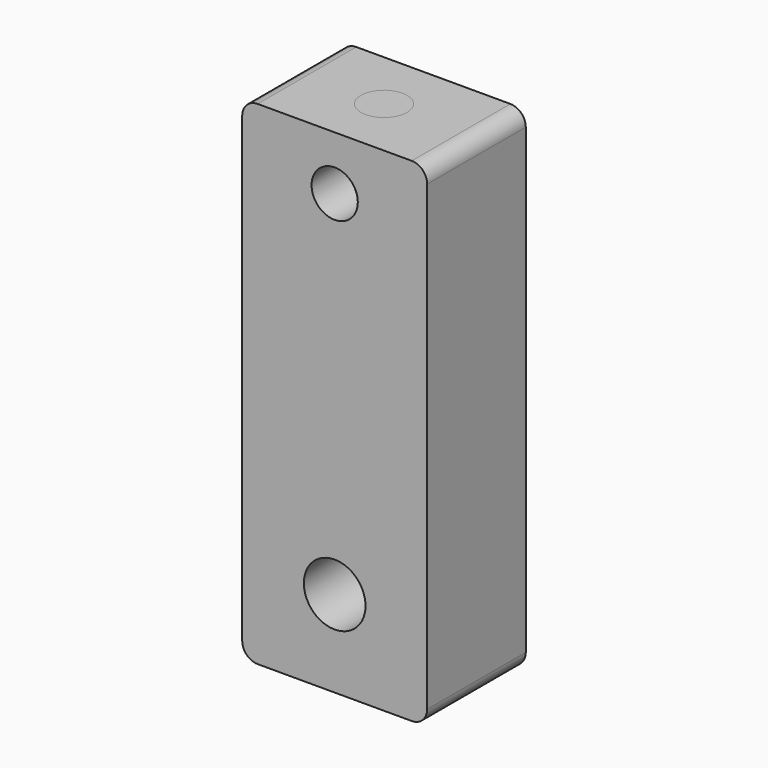
from build123d import *

# Parameters (mm, degrees)
F1_DEPTH = 25.4
F2_R     = 6.35
F3_DEPTH = 127
F4_R     = 4.7625
F5_DEPTH = 81.28
F7_R     = 4.7625
F8_DEPTH = 7.62
F6_R     = 4.7625
F9_DEPTH = 12.7


with BuildPart() as f1:
    # F0 (on Front) → F1 (new body)
    with BuildSketch(Plane.XZ):
        with BuildLine():
            ThreePointArc((0, 3.175), (0.9299359697, 0.9299359697), (3.175, 0))
            Line((3.175, 0), (34.925, 0))
            ThreePointArc((34.925, 0), (37.1700640303, 0.9299359697), (38.1, 3.175))
            Line((38.1, 3.175), (38.1, 98.425))
            ThreePointArc((38.1, 98.425), (37.1700640303, 100.6700640303), (34.925, 101.6))
            Line((34.925, 101.6), (3.175, 101.6))
            ThreePointArc((3.175, 101.6), (0.9299359697, 100.6700640303), (0, 98.425))
            Line((0, 98.425), (0, 3.175))
        make_face()
    extrude(amount=F1_DEPTH)

    # F2 (on face) → F3 (cut)
    with BuildSketch(Plane.XZ.offset(25.4)):
        with Locations((19.05, 17.78)):
            Circle(F2_R)
    extrude(amount=-F3_DEPTH, mode=Mode.SUBTRACT)

    # F4 (on face) → F5 (cut)
    with BuildSketch(Plane.XY.offset(101.6)):
        with Locations((19.05, -12.7)):
            Circle(F4_R)
    extrude(amount=-F5_DEPTH, mode=Mode.SUBTRACT)

    # F6 (on face) → F9 (cut)
    with BuildSketch(Plane.XZ.offset(25.4)):
        with Locations((19.05, 90.4875)):
            Circle(F6_R)
    extrude(amount=-F9_DEPTH, mode=Mode.SUBTRACT)


with BuildPart() as f8:
    # F7 (on face) → F8 (new body)
    with BuildSketch(Plane.XY.offset(101.6)):
        with Locations((19.05, -12.7)):
            Circle(F7_R)
    extrude(amount=-F8_DEPTH)


solid = Compound([f1.part, f8.part])
